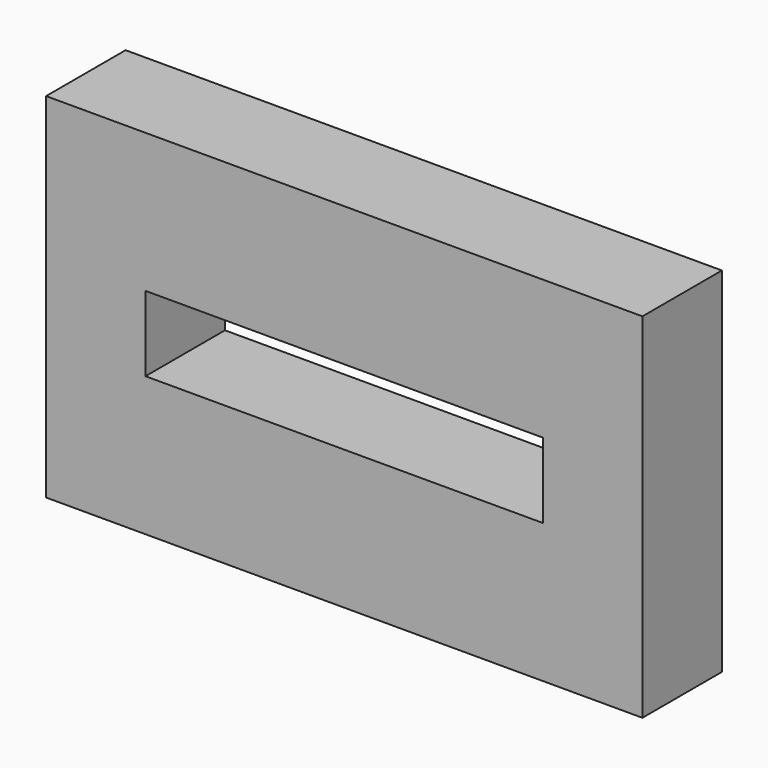
from build123d import *

# Parameters (mm, degrees)
F0_W     = 150
F0_H     = 88.9
F0_W_2   = 100
F0_H_2   = 18.9
F1_DEPTH = 25
F2_DEPTH = 190


# Not quite as in the source:
# - an extrude ends at something that could not be found from the text; its depth is read off the source's solid


with BuildPart() as f1:
    # F0 (on Front) → F1 (new body)
    with BuildSketch(Plane.XZ):
        with Locations((3.1299684197, -4.7291009414)):
            Rectangle(F0_W, F0_H)
        with Locations((3.1299684197, -4.7291009414)):
            Rectangle(F0_W_2, F0_H_2, mode=Mode.SUBTRACT)
    extrude(amount=F1_DEPTH)

    # F0 (on Front) → F2 (cut, through all)
    with BuildSketch(Plane.XZ):
        with Locations((3.1299684197, -4.7291009414)):
            Rectangle(F0_W_2, F0_H_2)
    extrude(amount=-F2_DEPTH, mode=Mode.SUBTRACT)


solid = f1.part
